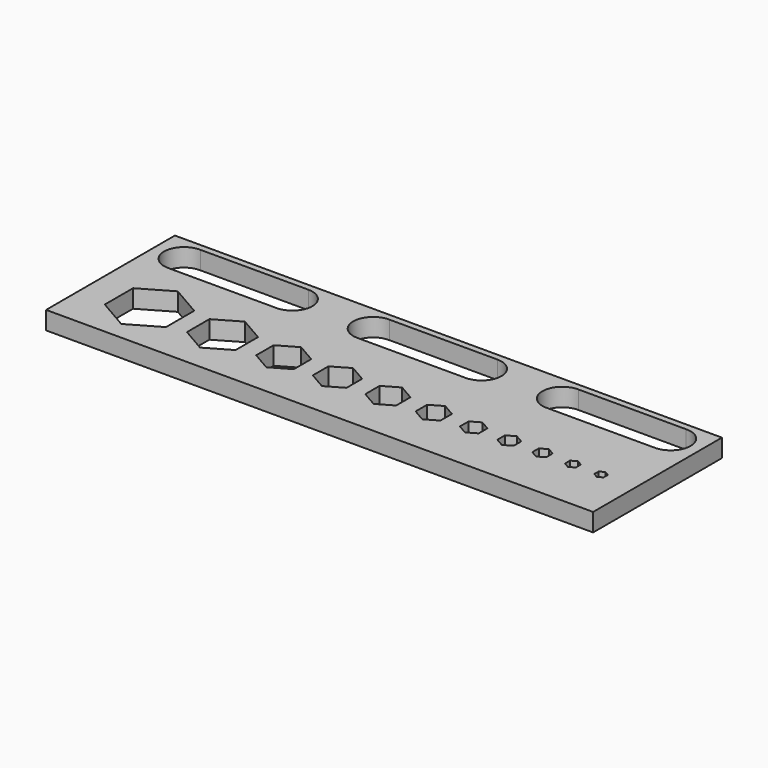
from build123d import *

# Parameters (mm, degrees)
F0_W     = 90.78
F0_H     = 17.7202104645
F1_DEPTH = 3
F3_D     = 6.6
F5_DEPTH = 25


with BuildPart() as f1:
    # F0 (on Top) → F1 (new body)
    with BuildSketch(Plane.XY):
        Polygon((-52.19, 13.3601052323), (-52.19, 8.8601052323), (38.59, 8.8601052323), (38.59, 13.3601052323), (38.59, 17.8601052323), (-52.19, 17.8601052323), align=None)
        with Locations((-6.8, 0)):
            Rectangle(F0_W, F0_H)
        Polygon((-42.115, 5.8601052323), (-37.04, 2.9300526161), (-37.04, -2.9300526161), (-42.115, -5.8601052323), (-47.19, -2.9300526161), (-47.19, 2.9300526161), align=None, mode=Mode.SUBTRACT)
        Polygon((-30.005, 4.6592166724), (-25.97, 2.3296083362), (-25.97, -2.3296083362), (-30.005, -4.6592166724), (-34.04, -2.3296083362), (-34.04, 2.3296083362), align=None, mode=Mode.SUBTRACT)
        Polygon((-19.845, 3.6084391824), (-16.72, 1.8042195912), (-16.72, -1.8042195912), (-19.845, -3.6084391824), (-22.97, -1.8042195912), (-22.97, 1.8042195912), align=None, mode=Mode.SUBTRACT)
        Polygon((-10.92, 3.2331615075), (-8.12, 1.6165807537), (-8.12, -1.6165807537), (-10.92, -3.2331615075), (-13.72, -1.6165807537), (-13.72, 1.6165807537), align=None, mode=Mode.SUBTRACT)
        Polygon((-2.56, 2.9560333783), (0, 1.4780166891), (0, -1.4780166891), (-2.56, -2.9560333783), (-5.12, -1.4780166891), (-5.12, 1.4780166891), align=None, mode=Mode.SUBTRACT)
        Polygon((5.06, 2.3786831091), (7.12, 1.1893415545), (7.12, -1.1893415545), (5.06, -2.3786831091), (3, -1.1893415545), (3, 1.1893415545), align=None, mode=Mode.SUBTRACT)
        Polygon((11.68, 1.8013328399), (13.24, 0.9006664199), (13.24, -0.9006664199), (11.68, -1.8013328399), (10.12, -0.9006664199), (10.12, 0.9006664199), align=None, mode=Mode.SUBTRACT)
        Polygon((17.595, 1.5646192295), (18.95, 0.7823096148), (18.95, -0.7823096148), (17.595, -1.5646192295), (16.24, -0.7823096148), (16.24, 0.7823096148), align=None, mode=Mode.SUBTRACT)
        Polygon((23.1, 1.3279056191), (24.25, 0.6639528096), (24.25, -0.6639528096), (23.1, -1.3279056191), (21.95, -0.6639528096), (21.95, 0.6639528096), align=None, mode=Mode.SUBTRACT)
        Polygon((28.15, 1.0392304845), (29.05, 0.5196152423), (29.05, -0.5196152423), (28.15, -1.0392304845), (27.25, -0.5196152423), (27.25, 0.5196152423), align=None, mode=Mode.SUBTRACT)
        Polygon((32.82, 0.8891194146), (33.59, 0.4445597073), (33.59, -0.4445597073), (32.82, -0.8891194146), (32.05, -0.4445597073), (32.05, 0.4445597073), align=None, mode=Mode.SUBTRACT)
    extrude(amount=F1_DEPTH)

    # F3 (through all)
    with Locations(Plane.XY.offset(3)):
        with Locations((-47.19, 13.4951905284), (-29.19, 13.4951905284), (-15.8, 13.4951905284), (2.2, 13.4951905284), (15.59, 13.4951905284), (33.59, 13.4951905284)):
            Hole(F3_D / 2)

    # F4 (on face) → F5 (cut)
    with BuildSketch(Plane.XY.offset(3)):
        with BuildLine():
            Line((-29.1901885501, 16.795190523), (-47.1078067859, 16.794166775))
            ThreePointArc((-47.1078067859, 16.794166775), (-44.8276666613, 15.79939998), (-43.89, 13.4951905284))
            ThreePointArc((-43.89, 13.4951905284), (-44.8276666613, 11.1909810768), (-47.1078067859, 10.1962142818))
            Line((-47.1078067859, 10.1962142818), (-29.1901885501, 10.1951905338))
            ThreePointArc((-29.1901885501, 10.1951905338), (-32.49, 13.4951905284), (-29.1901885501, 16.795190523))
        make_face()
        with BuildLine():
            Line((2.1994360639, 16.7951904802), (-15.7178067781, 16.7941667748))
            ThreePointArc((-15.7178067781, 16.7941667748), (-13.4376666586, 15.7993999772), (-12.5, 13.4951905284))
            ThreePointArc((-12.5, 13.4951905284), (-13.4377971224, 11.1908473324), (-15.7181803424, 10.1962049959))
            Line((-15.7181803424, 10.1962049959), (2.1998131641, 10.1951905337))
            ThreePointArc((2.1998131641, 10.1951905337), (-1.0999999946, 13.4950019783), (2.1994360639, 16.7951904802))
        make_face()
        with BuildLine():
            Line((33.5074298033, 16.794157361), (15.6725701967, 16.794157361))
            ThreePointArc((15.6725701967, 16.794157361), (17.9524649891, 15.799265001), (18.89, 13.4951905284))
            ThreePointArc((18.89, 13.4951905284), (17.9524649891, 11.1911160558), (15.6725701967, 10.1962236958))
            Line((15.6725701967, 10.1962236958), (33.4736921866, 10.1972407876))
            ThreePointArc((33.4736921866, 10.1972407876), (30.2900431541, 13.5120670006), (33.5074298033, 16.794157361))
        make_face()
    extrude(amount=-F5_DEPTH, mode=Mode.SUBTRACT)


solid = f1.part
